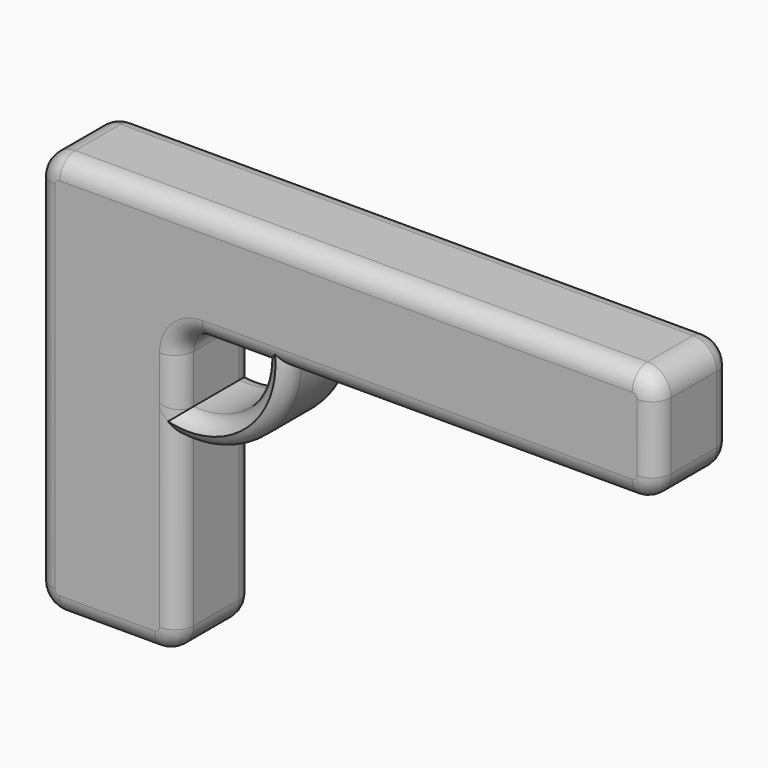
from build123d import *

# Parameters (mm, degrees)
F1_DEPTH      = 12.7
F2_T1_DEPTH   = 153.2337951016
F2_T3_DEPTH   = 95.3043418229
F2_T5_DEPTH   = 25.4
F2_T7_DEPTH   = 17.9600145107
F2_T10_ANGLE  = 90
F2_T12_ANGLE  = 90
F2_T14_ANGLE  = 90
F2_T18_DEPTH  = 58.0173112184
F2_S19_R      = 26.289
F2_T20_DEPTH  = 31
F2_T24_DEPTH  = 58.0173112184
F2_S25_R      = 20.32
F2_T26_DEPTH  = 31
F2_T30_ANGLE  = 149.8775603064
F2_T36_DEPTH  = 105.3526159376
F2_S37_R      = 20.32
F2_T38_DEPTH  = 54
F2_T42_DEPTH  = 105.3526159376
F2_S43_R      = 26.289
F2_T44_DEPTH  = 54
F2_T46_ANGLE  = 90
F2_T48_ANGLE  = 90
F2_T52_ANGLE  = 165.3398529119
F2_T58_DEPTH  = 25.6770160938
F2_S59_R      = 26.289
F2_T60_DEPTH  = 15
F2_T64_DEPTH  = 25.6770160938
F2_S65_R      = 20.32
F2_T66_DEPTH  = 15
F2_T68_ANGLE  = 90
F2_T72_DEPTH  = 28.831179164
F2_S73_R      = 20.32
F2_T74_DEPTH  = 16
F2_T78_DEPTH  = 28.831179164
F2_S79_R      = 26.289
F2_T80_DEPTH  = 16
F2_T82_ANGLE  = 90
F2_T84_ANGLE  = 90
F2_T86_ANGLE  = 90
F2_T90_DEPTH  = 58.0173112184
F2_S91_R      = 26.289
F2_T92_DEPTH  = 31
F2_T96_DEPTH  = 58.0173112184
F2_S97_R      = 20.32
F2_T98_DEPTH  = 31
F2_T102_ANGLE = 149.8775603064
F2_T108_DEPTH = 105.3526159376
F2_S109_R     = 20.32
F2_T110_DEPTH = 54
F2_T114_DEPTH = 105.3526159376
F2_S115_R     = 26.289
F2_T116_DEPTH = 54
F2_T118_ANGLE = 90
F2_T120_ANGLE = 90
F2_T124_ANGLE = 165.3398529119
F2_T130_DEPTH = 25.6770160938
F2_S131_R     = 26.289
F2_T132_DEPTH = 15
F2_T136_DEPTH = 25.6770160938
F2_S137_R     = 20.32
F2_T138_DEPTH = 15
F2_T140_ANGLE = 90
F2_T144_DEPTH = 28.831179164
F2_S145_R     = 20.32
F2_T146_DEPTH = 16
F2_T150_DEPTH = 28.831179164
F2_S151_R     = 26.289
F2_T152_DEPTH = 16
F2_T157_ANGLE = 149.8775603064
F2_T161_DEPTH = 58.0173112184
F2_S162_R     = 26.289
F2_T163_DEPTH = 31
F2_S164_R     = 20.32
F2_T165_DEPTH = 31
F2_T171_DEPTH = 105.3526159376
F2_S172_R     = 26.289
F2_T173_DEPTH = 54
F2_S174_R     = 20.32
F2_T175_DEPTH = 54
F2_T178_ANGLE = 149.8775603064
F2_T185_ANGLE = 165.3398529119
F2_T189_DEPTH = 28.831179164
F2_S190_R     = 26.289
F2_T191_DEPTH = 16
F2_S192_R     = 20.32
F2_T193_DEPTH = 16
F2_T199_ANGLE = 165.3398529119
F2_T203_DEPTH = 25.6770160938
F2_S204_R     = 26.289
F2_T205_DEPTH = 15
F2_S206_R     = 20.32
F2_T207_DEPTH = 15
F2_T213_ANGLE = 149.8775603064
F2_T217_DEPTH = 58.0173112184
F2_S218_R     = 26.289
F2_T219_DEPTH = 31
F2_S220_R     = 20.32
F2_T221_DEPTH = 31
F2_T227_DEPTH = 105.3526159376
F2_S228_R     = 26.289
F2_T229_DEPTH = 54
F2_S230_R     = 20.32
F2_T231_DEPTH = 54
F2_T234_ANGLE = 149.8775603064
F2_T241_DEPTH = 28.831179164
F2_S242_R     = 26.289
F2_T243_DEPTH = 16
F2_S244_R     = 20.32
F2_T245_DEPTH = 16
F2_T248_ANGLE = 165.3398529119
F2_T255_DEPTH = 25.6770160938
F2_S256_R     = 26.289
F2_T257_DEPTH = 15
F2_S258_R     = 20.32
F2_T259_DEPTH = 15
F2_T262_ANGLE = 165.3398529119


# Not quite as in the source:
# - a fillet or chamfer that OpenCascade refuses, or shapes differently, is made with other operations: its cross-section is extruded or revolved along the edge and cut away or added


with BuildPart() as f1:
    # F0 (on Front) → F1 (new body, symmetric)
    with BuildSketch(Plane.XZ):
        with BuildLine():
            Line((-31.75, -76.2), (-6.35, -76.2))
            ThreePointArc((-6.35, -76.2), (-1.8598719395, -74.3401280605), (0, -69.85))
            Line((0, -69.85), (0, -24.5326887816))
            ThreePointArc((0, -24.5326887816), (20.0309214376, -17.9992996084), (28.831179164, 1.1443273122))
            Line((28.831179164, 1.1443273122), (121.4837951016, 1.1443273122))
            ThreePointArc((121.4837951016, 1.1443273122), (125.9739231621, 3.0041992516), (127.8337951016, 7.4943273122))
            Line((127.8337951016, 7.4943273122), (127.8337951016, 25.4543418229))
            ThreePointArc((127.8337951016, 25.4543418229), (125.9739231621, 29.9444698834), (121.4837951016, 31.8043418229))
            Line((121.4837951016, 31.8043418229), (-31.75, 31.8043418229))
            ThreePointArc((-31.75, 31.8043418229), (-36.2401280605, 29.9444698834), (-38.1, 25.4543418229))
            Line((-38.1, 25.4543418229), (-38.1, -69.85))
            ThreePointArc((-38.1, -69.85), (-36.2401280605, -74.3401280605), (-31.75, -76.2))
        make_face()
        with BuildLine():
            Line((0, -18.1826887816), (0, -5.2056726878))
            ThreePointArc((0, -5.2056726878), (1.8598719395, -0.7155446273), (6.35, 1.1443273122))
            Line((6.35, 1.1443273122), (22.481179164, 1.1443273122))
            ThreePointArc((22.481179164, 1.1443273122), (15.4268166396, -13.3885987579), (0, -18.1826887816))
        make_face(mode=Mode.SUBTRACT)
    extrude(amount=F1_DEPTH, both=True)

    # F2: fillet of radius 5.08 on 32 edges, made by hand

    # F2_s2 → F2_t1 (cut)
    with BuildSketch(Plane.YZ.offset(-31.75)):
        with BuildLine():
            ThreePointArc((-7.62, 31.8043418229), (-11.2121024484, 30.3164442713), (-12.7, 26.7243418229))
            Line((-12.7, 26.7243418229), (-12.7, 31.8043418229))
            Line((-12.7, 31.8043418229), (-7.62, 31.8043418229))
        make_face()
        with BuildLine():
            ThreePointArc((7.62, 31.8043418229), (11.2121024484, 30.3164442713), (12.7, 26.7243418229))
            Line((12.7, 26.7243418229), (12.7, 31.8043418229))
            Line((12.7, 31.8043418229), (7.62, 31.8043418229))
        make_face()
    extrude(amount=F2_T1_DEPTH, mode=Mode.SUBTRACT)

    # F2_s4 → F2_t3 (cut)
    with BuildSketch(Plane.XY.offset(-69.85)):
        with BuildLine():
            ThreePointArc((-38.1, -7.62), (-36.6121024484, -11.2121024484), (-33.02, -12.7))
            Line((-33.02, -12.7), (-38.1, -12.7))
            Line((-38.1, -12.7), (-38.1, -7.62))
        make_face()
        with BuildLine():
            ThreePointArc((-38.1, 7.62), (-36.6121024484, 11.2121024484), (-33.02, 12.7))
            Line((-33.02, 12.7), (-38.1, 12.7))
            Line((-38.1, 12.7), (-38.1, 7.62))
        make_face()
    extrude(amount=F2_T3_DEPTH, mode=Mode.SUBTRACT)

    # F2_s6 → F2_t5 (cut)
    with BuildSketch(Plane.YZ.offset(-31.75)):
        with BuildLine():
            ThreePointArc((-7.62, -76.2), (-11.2121024484, -74.7121024484), (-12.7, -71.12))
            Line((-12.7, -71.12), (-12.7, -76.2))
            Line((-12.7, -76.2), (-7.62, -76.2))
        make_face()
        with BuildLine():
            ThreePointArc((7.62, -76.2), (11.2121024484, -74.7121024484), (12.7, -71.12))
            Line((12.7, -71.12), (12.7, -76.2))
            Line((12.7, -76.2), (7.62, -76.2))
        make_face()
    extrude(amount=F2_T5_DEPTH, mode=Mode.SUBTRACT)

    # F2_s8 → F2_t7 (cut)
    with BuildSketch(Plane.XY.offset(7.4943273122)):
        with BuildLine():
            ThreePointArc((127.8337951016, -7.62), (126.34589755, -11.2121024484), (122.7537951016, -12.7))
            Line((122.7537951016, -12.7), (127.8337951016, -12.7))
            Line((127.8337951016, -12.7), (127.8337951016, -7.62))
        make_face()
        with BuildLine():
            ThreePointArc((127.8337951016, 7.62), (126.34589755, 11.2121024484), (122.7537951016, 12.7))
            Line((122.7537951016, 12.7), (127.8337951016, 12.7))
            Line((127.8337951016, 12.7), (127.8337951016, 7.62))
        make_face()
    extrude(amount=F2_T7_DEPTH, mode=Mode.SUBTRACT)

    # F2_s9 → F2_t10 (revolve, cut)
    with BuildSketch(Plane.YZ.offset(-31.75)):
        with BuildLine():
            ThreePointArc((-12.7, 26.7243418229), (-11.2121024484, 30.3164442713), (-7.62, 31.8043418229))
            Line((-7.62, 31.8043418229), (-12.7, 31.8043418229))
            Line((-12.7, 31.8043418229), (-12.7, 26.7243418229))
        make_face()
    revolve(axis=Axis((-31.75, -12.7, 25.4543418229), (0, -1, 0)), revolution_arc=F2_T10_ANGLE, mode=Mode.SUBTRACT)

    # F2_s11 → F2_t12 (revolve, cut)
    with BuildSketch(Plane.XY.offset(-69.85)):
        with BuildLine():
            ThreePointArc((-38.1, -7.62), (-36.6121024484, -11.2121024484), (-33.02, -12.7))
            Line((-33.02, -12.7), (-38.1, -12.7))
            Line((-38.1, -12.7), (-38.1, -7.62))
        make_face()
    revolve(axis=Axis((-31.75, -12.7, -69.85), (0, -1, 0)), revolution_arc=F2_T12_ANGLE, mode=Mode.SUBTRACT)

    # F2_s13 → F2_t14 (revolve, cut)
    with BuildSketch(Plane.YZ.offset(-6.35)):
        with BuildLine():
            ThreePointArc((-7.62, -76.2), (-11.2121024484, -74.7121024484), (-12.7, -71.12))
            Line((-12.7, -71.12), (-12.7, -76.2))
            Line((-12.7, -76.2), (-7.62, -76.2))
        make_face()
    revolve(axis=Axis((-6.35, -12.7, -69.85), (0, -1, 0)), revolution_arc=F2_T14_ANGLE, mode=Mode.SUBTRACT)


with BuildPart() as f2_tool16:
    # F2_s17 → F2_t18 (new body)
    with BuildSketch(Plane.XY.offset(-69.85)):
        with BuildLine():
            ThreePointArc((0, -7.62), (-1.4878975516, -11.2121024484), (-5.08, -12.7))
            Line((-5.08, -12.7), (0, -12.7))
            Line((0, -12.7), (0, -7.62))
        make_face()
    extrude(amount=F2_T18_DEPTH)

    # F2_s19 → F2_t20 (cut, symmetric)
    with BuildSketch(Plane.XZ.offset(10.2)):
        with Locations((2.5467151815, 1.6326654637)):
            Circle(F2_S19_R)
    extrude(amount=F2_T20_DEPTH, both=True, mode=Mode.SUBTRACT)


with BuildPart() as f1_1:
    add(f1.part)

    # F2_t15: cut F2_tool16
    add(f2_tool16.part, mode=Mode.SUBTRACT)


with BuildPart() as f2_tool22:
    # F2_s23 → F2_t24 (new body)
    with BuildSketch(Plane.XY.offset(-69.85)):
        with BuildLine():
            ThreePointArc((0, -7.62), (-1.4878975516, -11.2121024484), (-5.08, -12.7))
            Line((-5.08, -12.7), (0, -12.7))
            Line((0, -12.7), (0, -7.62))
        make_face()
    extrude(amount=F2_T24_DEPTH)

    # F2_s25 → F2_t26 (intersect, symmetric)
    with BuildSketch(Plane.XZ.offset(10.2)):
        with Locations((2.1800572993, 2.0200276241)):
            Circle(F2_S25_R)
    extrude(amount=F2_T26_DEPTH, both=True, mode=Mode.INTERSECT)


with BuildPart() as f1_2:
    add(f1_1.part)

    # F2_t21: cut F2_tool22
    add(f2_tool22.part, mode=Mode.SUBTRACT)


with BuildPart() as f2_tool28:
    # F2_s29 → F2_t30 (revolve)
    with BuildSketch(Plane(origin=(1.0324526072, 0, -0.6769199165), x_dir=(0, 1, 0), z_dir=(-0.8362808351, 0, 0.5483013449))):
        with BuildLine():
            ThreePointArc((-7.62, 23.5272658034), (-11.2121024484, 22.0393682518), (-12.7, 18.4472658034))
            Line((-12.7, 18.4472658034), (-12.7, 23.5272658034))
            Line((-12.7, 23.5272658034), (-7.62, 23.5272658034))
        make_face()
    revolve(axis=Axis((2.5467151815, -12.7, 1.6326654637), (0, -1, 0)), revolution_arc=F2_T30_ANGLE)

    split(bisect_by=Plane.XY.offset(1.1443273122), keep=Keep.BOTTOM)

    split(bisect_by=Plane.YZ, keep=Keep.TOP)


with BuildPart() as f1_3:
    add(f1_2.part)

    # F2_t27: cut F2_tool28
    add(f2_tool28.part, mode=Mode.SUBTRACT)


with BuildPart() as f2_tool34:
    # F2_s35 → F2_t36 (new body)
    with BuildSketch(Plane.YZ.offset(16.131179164)):
        with BuildLine():
            ThreePointArc((-7.62, 1.1443273122), (-11.2121024484, 2.6322248637), (-12.7, 6.2243273122))
            Line((-12.7, 6.2243273122), (-12.7, 1.1443273122))
            Line((-12.7, 1.1443273122), (-7.62, 1.1443273122))
        make_face()
    extrude(amount=F2_T36_DEPTH)

    # F2_s37 → F2_t38 (intersect, symmetric)
    with BuildSketch(Plane.XZ.offset(10.2)):
        with Locations((2.1800572993, 2.0200276241)):
            Circle(F2_S37_R)
    extrude(amount=F2_T38_DEPTH, both=True, mode=Mode.INTERSECT)


with BuildPart() as f1_4:
    add(f1_3.part)

    # F2_t33: cut F2_tool34
    add(f2_tool34.part, mode=Mode.SUBTRACT)


with BuildPart() as f2_tool40:
    # F2_s41 → F2_t42 (new body)
    with BuildSketch(Plane.YZ.offset(16.131179164)):
        with BuildLine():
            ThreePointArc((-7.62, 1.1443273122), (-11.2121024484, 2.6322248637), (-12.7, 6.2243273122))
            Line((-12.7, 6.2243273122), (-12.7, 1.1443273122))
            Line((-12.7, 1.1443273122), (-7.62, 1.1443273122))
        make_face()
    extrude(amount=F2_T42_DEPTH)

    # F2_s43 → F2_t44 (cut, symmetric)
    with BuildSketch(Plane.XZ.offset(10.2)):
        with Locations((2.5467151815, 1.6326654637)):
            Circle(F2_S43_R)
    extrude(amount=F2_T44_DEPTH, both=True, mode=Mode.SUBTRACT)


with BuildPart() as f1_5:
    add(f1_4.part)

    # F2_t39: cut F2_tool40
    add(f2_tool40.part, mode=Mode.SUBTRACT)

    # F2_s45 → F2_t46 (revolve, cut)
    with BuildSketch(Plane.YZ.offset(121.4837951016)):
        with BuildLine():
            ThreePointArc((-7.62, 1.1443273122), (-11.2121024484, 2.6322248637), (-12.7, 6.2243273122))
            Line((-12.7, 6.2243273122), (-12.7, 1.1443273122))
            Line((-12.7, 1.1443273122), (-7.62, 1.1443273122))
        make_face()
    revolve(axis=Axis((121.4837951016, -12.7, 7.4943273122), (0, -1, 0)), revolution_arc=F2_T46_ANGLE, mode=Mode.SUBTRACT)

    # F2_s47 → F2_t48 (revolve, cut)
    with BuildSketch(Plane.XY.offset(25.4543418229)):
        with BuildLine():
            ThreePointArc((127.8337951016, -7.62), (126.34589755, -11.2121024484), (122.7537951016, -12.7))
            Line((122.7537951016, -12.7), (127.8337951016, -12.7))
            Line((127.8337951016, -12.7), (127.8337951016, -7.62))
        make_face()
    revolve(axis=Axis((121.4837951016, -12.7, 25.4543418229), (0, -1, 0)), revolution_arc=F2_T48_ANGLE, mode=Mode.SUBTRACT)


with BuildPart() as f2_tool50:
    # F2_s51 → F2_t52 (revolve)
    with BuildSketch(Plane(origin=(-0.2686553541, 0, 0.4081266668), x_dir=(0, 1, 0), z_dir=(-0.5498321217, 0, 0.835275187))):
        with BuildLine():
            ThreePointArc((-12.7, -28.3316238427), (-11.2121024484, -24.7395213943), (-7.62, -23.2516238427))
            Line((-7.62, -23.2516238427), (-12.7, -23.2516238427))
            Line((-12.7, -23.2516238427), (-12.7, -28.3316238427))
        make_face()
    revolve(axis=Axis((2.1800572993, -12.7, 2.0200276241), (0, 1, 0)), revolution_arc=F2_T52_ANGLE)

    split(bisect_by=Plane.XY.offset(1.1443273122), keep=Keep.BOTTOM)

    split(bisect_by=Plane.YZ, keep=Keep.TOP)


with BuildPart() as f1_6:
    add(f1_5.part)

    # F2_t49: cut F2_tool50
    add(f2_tool50.part, mode=Mode.SUBTRACT)


with BuildPart() as f2_tool56:
    # F2_s57 → F2_t58 (new body)
    with BuildSketch(Plane.XY.offset(-30.8826887816)):
        with BuildLine():
            ThreePointArc((-5.08, -12.7), (-1.4878975516, -11.2121024484), (0, -7.62))
            Line((0, -7.62), (0, -12.7))
            Line((0, -12.7), (-5.08, -12.7))
        make_face()
    extrude(amount=F2_T58_DEPTH)

    # F2_s59 → F2_t60 (cut, symmetric)
    with BuildSketch(Plane.XZ.offset(10.2)):
        with Locations((2.5467151815, 1.6326654637)):
            Circle(F2_S59_R)
    extrude(amount=F2_T60_DEPTH, both=True, mode=Mode.SUBTRACT)


with BuildPart() as f1_7:
    add(f1_6.part)

    # F2_t55: cut F2_tool56
    add(f2_tool56.part, mode=Mode.SUBTRACT)


with BuildPart() as f2_tool62:
    # F2_s63 → F2_t64 (new body)
    with BuildSketch(Plane.XY.offset(-30.8826887816)):
        with BuildLine():
            ThreePointArc((-5.08, -12.7), (-1.4878975516, -11.2121024484), (0, -7.62))
            Line((0, -7.62), (0, -12.7))
            Line((0, -12.7), (-5.08, -12.7))
        make_face()
    extrude(amount=F2_T64_DEPTH)

    # F2_s65 → F2_t66 (intersect, symmetric)
    with BuildSketch(Plane.XZ.offset(10.2)):
        with Locations((2.1800572993, 2.0200276241)):
            Circle(F2_S65_R)
    extrude(amount=F2_T66_DEPTH, both=True, mode=Mode.INTERSECT)


with BuildPart() as f1_8:
    add(f1_7.part)

    # F2_t61: cut F2_tool62
    add(f2_tool62.part, mode=Mode.SUBTRACT)

    # F2_s67 → F2_t68 (revolve, cut)
    with BuildSketch(Plane.XY.offset(-5.2056726878)):
        with BuildLine():
            ThreePointArc((-5.08, -12.7), (-1.4878975516, -11.2121024484), (0, -7.62))
            Line((0, -7.62), (0, -12.7))
            Line((0, -12.7), (-5.08, -12.7))
        make_face()
    revolve(axis=Axis((6.35, -12.7, -5.2056726878), (0, 1, 0)), revolution_arc=F2_T68_ANGLE, mode=Mode.SUBTRACT)


with BuildPart() as f2_tool70:
    # F2_s71 → F2_t72 (new body)
    with BuildSketch(Plane.YZ.offset(6.35)):
        with BuildLine():
            ThreePointArc((-12.7, 6.2243273122), (-11.2121024484, 2.6322248637), (-7.62, 1.1443273122))
            Line((-7.62, 1.1443273122), (-12.7, 1.1443273122))
            Line((-12.7, 1.1443273122), (-12.7, 6.2243273122))
        make_face()
    extrude(amount=F2_T72_DEPTH)

    # F2_s73 → F2_t74 (intersect, symmetric)
    with BuildSketch(Plane.XZ.offset(10.2)):
        with Locations((2.1800572993, 2.0200276241)):
            Circle(F2_S73_R)
    extrude(amount=F2_T74_DEPTH, both=True, mode=Mode.INTERSECT)


with BuildPart() as f1_9:
    add(f1_8.part)

    # F2_t69: cut F2_tool70
    add(f2_tool70.part, mode=Mode.SUBTRACT)


with BuildPart() as f2_tool76:
    # F2_s77 → F2_t78 (new body)
    with BuildSketch(Plane.YZ.offset(6.35)):
        with BuildLine():
            ThreePointArc((-12.7, 6.2243273122), (-11.2121024484, 2.6322248637), (-7.62, 1.1443273122))
            Line((-7.62, 1.1443273122), (-12.7, 1.1443273122))
            Line((-12.7, 1.1443273122), (-12.7, 6.2243273122))
        make_face()
    extrude(amount=F2_T78_DEPTH)

    # F2_s79 → F2_t80 (cut, symmetric)
    with BuildSketch(Plane.XZ.offset(10.2)):
        with Locations((2.5467151815, 1.6326654637)):
            Circle(F2_S79_R)
    extrude(amount=F2_T80_DEPTH, both=True, mode=Mode.SUBTRACT)


with BuildPart() as f1_10:
    add(f1_9.part)

    # F2_t75: cut F2_tool76
    add(f2_tool76.part, mode=Mode.SUBTRACT)

    # F2_s81 → F2_t82 (revolve, cut)
    with BuildSketch(Plane.YZ.offset(-31.75)):
        with BuildLine():
            ThreePointArc((7.62, 31.8043418229), (11.2121024484, 30.3164442713), (12.7, 26.7243418229))
            Line((12.7, 26.7243418229), (12.7, 31.8043418229))
            Line((12.7, 31.8043418229), (7.62, 31.8043418229))
        make_face()
    revolve(axis=Axis((-31.75, 12.7, 25.4543418229), (0, -1, 0)), revolution_arc=F2_T82_ANGLE, mode=Mode.SUBTRACT)

    # F2_s83 → F2_t84 (revolve, cut)
    with BuildSketch(Plane.XY.offset(-69.85)):
        with BuildLine():
            ThreePointArc((-38.1, 7.62), (-36.6121024484, 11.2121024484), (-33.02, 12.7))
            Line((-33.02, 12.7), (-38.1, 12.7))
            Line((-38.1, 12.7), (-38.1, 7.62))
        make_face()
    revolve(axis=Axis((-31.75, 12.7, -69.85), (0, -1, 0)), revolution_arc=F2_T84_ANGLE, mode=Mode.SUBTRACT)

    # F2_s85 → F2_t86 (revolve, cut)
    with BuildSketch(Plane.YZ.offset(-6.35)):
        with BuildLine():
            ThreePointArc((7.62, -76.2), (11.2121024484, -74.7121024484), (12.7, -71.12))
            Line((12.7, -71.12), (12.7, -76.2))
            Line((12.7, -76.2), (7.62, -76.2))
        make_face()
    revolve(axis=Axis((-6.35, 12.7, -69.85), (0, -1, 0)), revolution_arc=F2_T86_ANGLE, mode=Mode.SUBTRACT)


with BuildPart() as f2_tool88:
    # F2_s89 → F2_t90 (new body)
    with BuildSketch(Plane.XY.offset(-69.85)):
        with BuildLine():
            ThreePointArc((0, 7.62), (-1.4878975516, 11.2121024484), (-5.08, 12.7))
            Line((-5.08, 12.7), (0, 12.7))
            Line((0, 12.7), (0, 7.62))
        make_face()
    extrude(amount=F2_T90_DEPTH)

    # F2_s91 → F2_t92 (cut, symmetric)
    with BuildSketch(Plane.XZ.offset(-10.2)):
        with Locations((2.5467151815, 1.6326654637)):
            Circle(F2_S91_R)
    extrude(amount=F2_T92_DEPTH, both=True, mode=Mode.SUBTRACT)


with BuildPart() as f1_11:
    add(f1_10.part)

    # F2_t87: cut F2_tool88
    add(f2_tool88.part, mode=Mode.SUBTRACT)


with BuildPart() as f2_tool94:
    # F2_s95 → F2_t96 (new body)
    with BuildSketch(Plane.XY.offset(-69.85)):
        with BuildLine():
            ThreePointArc((0, 7.62), (-1.4878975516, 11.2121024484), (-5.08, 12.7))
            Line((-5.08, 12.7), (0, 12.7))
            Line((0, 12.7), (0, 7.62))
        make_face()
    extrude(amount=F2_T96_DEPTH)

    # F2_s97 → F2_t98 (intersect, symmetric)
    with BuildSketch(Plane.XZ.offset(-10.2)):
        with Locations((2.1800572993, 2.0200276241)):
            Circle(F2_S97_R)
    extrude(amount=F2_T98_DEPTH, both=True, mode=Mode.INTERSECT)


with BuildPart() as f1_12:
    add(f1_11.part)

    # F2_t93: cut F2_tool94
    add(f2_tool94.part, mode=Mode.SUBTRACT)


with BuildPart() as f2_tool100:
    # F2_s101 → F2_t102 (revolve)
    with BuildSketch(Plane(origin=(1.0324526072, 0, -0.6769199165), x_dir=(0, 1, 0), z_dir=(-0.8362808351, 0, 0.5483013449))):
        with BuildLine():
            ThreePointArc((7.62, 23.5272658034), (11.2121024484, 22.0393682518), (12.7, 18.4472658034))
            Line((12.7, 18.4472658034), (12.7, 23.5272658034))
            Line((12.7, 23.5272658034), (7.62, 23.5272658034))
        make_face()
    revolve(axis=Axis((2.5467151815, 12.7, 1.6326654637), (0, -1, 0)), revolution_arc=F2_T102_ANGLE)

    split(bisect_by=Plane.XY.offset(1.1443273122), keep=Keep.BOTTOM)

    split(bisect_by=Plane.YZ, keep=Keep.TOP)


with BuildPart() as f1_13:
    add(f1_12.part)

    # F2_t99: cut F2_tool100
    add(f2_tool100.part, mode=Mode.SUBTRACT)


with BuildPart() as f2_tool106:
    # F2_s107 → F2_t108 (new body)
    with BuildSketch(Plane.YZ.offset(16.131179164)):
        with BuildLine():
            ThreePointArc((7.62, 1.1443273122), (11.2121024484, 2.6322248637), (12.7, 6.2243273122))
            Line((12.7, 6.2243273122), (12.7, 1.1443273122))
            Line((12.7, 1.1443273122), (7.62, 1.1443273122))
        make_face()
    extrude(amount=F2_T108_DEPTH)

    # F2_s109 → F2_t110 (intersect, symmetric)
    with BuildSketch(Plane.XZ.offset(-10.2)):
        with Locations((2.1800572993, 2.0200276241)):
            Circle(F2_S109_R)
    extrude(amount=F2_T110_DEPTH, both=True, mode=Mode.INTERSECT)


with BuildPart() as f1_14:
    add(f1_13.part)

    # F2_t105: cut F2_tool106
    add(f2_tool106.part, mode=Mode.SUBTRACT)


with BuildPart() as f2_tool112:
    # F2_s113 → F2_t114 (new body)
    with BuildSketch(Plane.YZ.offset(16.131179164)):
        with BuildLine():
            ThreePointArc((7.62, 1.1443273122), (11.2121024484, 2.6322248637), (12.7, 6.2243273122))
            Line((12.7, 6.2243273122), (12.7, 1.1443273122))
            Line((12.7, 1.1443273122), (7.62, 1.1443273122))
        make_face()
    extrude(amount=F2_T114_DEPTH)

    # F2_s115 → F2_t116 (cut, symmetric)
    with BuildSketch(Plane.XZ.offset(-10.2)):
        with Locations((2.5467151815, 1.6326654637)):
            Circle(F2_S115_R)
    extrude(amount=F2_T116_DEPTH, both=True, mode=Mode.SUBTRACT)


with BuildPart() as f1_15:
    add(f1_14.part)

    # F2_t111: cut F2_tool112
    add(f2_tool112.part, mode=Mode.SUBTRACT)

    # F2_s117 → F2_t118 (revolve, cut)
    with BuildSketch(Plane.YZ.offset(121.4837951016)):
        with BuildLine():
            ThreePointArc((7.62, 1.1443273122), (11.2121024484, 2.6322248637), (12.7, 6.2243273122))
            Line((12.7, 6.2243273122), (12.7, 1.1443273122))
            Line((12.7, 1.1443273122), (7.62, 1.1443273122))
        make_face()
    revolve(axis=Axis((121.4837951016, 12.7, 7.4943273122), (0, -1, 0)), revolution_arc=F2_T118_ANGLE, mode=Mode.SUBTRACT)

    # F2_s119 → F2_t120 (revolve, cut)
    with BuildSketch(Plane.XY.offset(25.4543418229)):
        with BuildLine():
            ThreePointArc((127.8337951016, 7.62), (126.34589755, 11.2121024484), (122.7537951016, 12.7))
            Line((122.7537951016, 12.7), (127.8337951016, 12.7))
            Line((127.8337951016, 12.7), (127.8337951016, 7.62))
        make_face()
    revolve(axis=Axis((121.4837951016, 12.7, 25.4543418229), (0, -1, 0)), revolution_arc=F2_T120_ANGLE, mode=Mode.SUBTRACT)


with BuildPart() as f2_tool122:
    # F2_s123 → F2_t124 (revolve)
    with BuildSketch(Plane(origin=(-0.2686553541, 0, 0.4081266668), x_dir=(0, 1, 0), z_dir=(-0.5498321217, 0, 0.835275187))):
        with BuildLine():
            ThreePointArc((7.62, -23.2516238427), (11.2121024484, -24.7395213943), (12.7, -28.3316238427))
            Line((12.7, -28.3316238427), (12.7, -23.2516238427))
            Line((12.7, -23.2516238427), (7.62, -23.2516238427))
        make_face()
    revolve(axis=Axis((2.1800572993, 12.7, 2.0200276241), (0, 1, 0)), revolution_arc=F2_T124_ANGLE)

    split(bisect_by=Plane.XY.offset(1.1443273122), keep=Keep.BOTTOM)

    split(bisect_by=Plane.YZ, keep=Keep.TOP)


with BuildPart() as f1_16:
    add(f1_15.part)

    # F2_t121: cut F2_tool122
    add(f2_tool122.part, mode=Mode.SUBTRACT)


with BuildPart() as f2_tool128:
    # F2_s129 → F2_t130 (new body)
    with BuildSketch(Plane.XY.offset(-30.8826887816)):
        with BuildLine():
            ThreePointArc((0, 7.62), (-1.4878975516, 11.2121024484), (-5.08, 12.7))
            Line((-5.08, 12.7), (0, 12.7))
            Line((0, 12.7), (0, 7.62))
        make_face()
    extrude(amount=F2_T130_DEPTH)

    # F2_s131 → F2_t132 (cut, symmetric)
    with BuildSketch(Plane.XZ.offset(-10.2)):
        with Locations((2.5467151815, 1.6326654637)):
            Circle(F2_S131_R)
    extrude(amount=F2_T132_DEPTH, both=True, mode=Mode.SUBTRACT)


with BuildPart() as f1_17:
    add(f1_16.part)

    # F2_t127: cut F2_tool128
    add(f2_tool128.part, mode=Mode.SUBTRACT)


with BuildPart() as f2_tool134:
    # F2_s135 → F2_t136 (new body)
    with BuildSketch(Plane.XY.offset(-30.8826887816)):
        with BuildLine():
            ThreePointArc((0, 7.62), (-1.4878975516, 11.2121024484), (-5.08, 12.7))
            Line((-5.08, 12.7), (0, 12.7))
            Line((0, 12.7), (0, 7.62))
        make_face()
    extrude(amount=F2_T136_DEPTH)

    # F2_s137 → F2_t138 (intersect, symmetric)
    with BuildSketch(Plane.XZ.offset(-10.2)):
        with Locations((2.1800572993, 2.0200276241)):
            Circle(F2_S137_R)
    extrude(amount=F2_T138_DEPTH, both=True, mode=Mode.INTERSECT)


with BuildPart() as f1_18:
    add(f1_17.part)

    # F2_t133: cut F2_tool134
    add(f2_tool134.part, mode=Mode.SUBTRACT)

    # F2_s139 → F2_t140 (revolve, cut)
    with BuildSketch(Plane.XY.offset(-5.2056726878)):
        with BuildLine():
            ThreePointArc((0, 7.62), (-1.4878975516, 11.2121024484), (-5.08, 12.7))
            Line((-5.08, 12.7), (0, 12.7))
            Line((0, 12.7), (0, 7.62))
        make_face()
    revolve(axis=Axis((6.35, 12.7, -5.2056726878), (0, 1, 0)), revolution_arc=F2_T140_ANGLE, mode=Mode.SUBTRACT)


with BuildPart() as f2_tool142:
    # F2_s143 → F2_t144 (new body)
    with BuildSketch(Plane.YZ.offset(6.35)):
        with BuildLine():
            ThreePointArc((7.62, 1.1443273122), (11.2121024484, 2.6322248637), (12.7, 6.2243273122))
            Line((12.7, 6.2243273122), (12.7, 1.1443273122))
            Line((12.7, 1.1443273122), (7.62, 1.1443273122))
        make_face()
    extrude(amount=F2_T144_DEPTH)

    # F2_s145 → F2_t146 (intersect, symmetric)
    with BuildSketch(Plane.XZ.offset(-10.2)):
        with Locations((2.1800572993, 2.0200276241)):
            Circle(F2_S145_R)
    extrude(amount=F2_T146_DEPTH, both=True, mode=Mode.INTERSECT)


with BuildPart() as f1_19:
    add(f1_18.part)

    # F2_t141: cut F2_tool142
    add(f2_tool142.part, mode=Mode.SUBTRACT)


with BuildPart() as f2_tool148:
    # F2_s149 → F2_t150 (new body)
    with BuildSketch(Plane.YZ.offset(6.35)):
        with BuildLine():
            ThreePointArc((7.62, 1.1443273122), (11.2121024484, 2.6322248637), (12.7, 6.2243273122))
            Line((12.7, 6.2243273122), (12.7, 1.1443273122))
            Line((12.7, 1.1443273122), (7.62, 1.1443273122))
        make_face()
    extrude(amount=F2_T150_DEPTH)

    # F2_s151 → F2_t152 (cut, symmetric)
    with BuildSketch(Plane.XZ.offset(-10.2)):
        with Locations((2.5467151815, 1.6326654637)):
            Circle(F2_S151_R)
    extrude(amount=F2_T152_DEPTH, both=True, mode=Mode.SUBTRACT)


with BuildPart() as f1_20:
    add(f1_19.part)

    # F2_t147: cut F2_tool148
    add(f2_tool148.part, mode=Mode.SUBTRACT)


with BuildPart() as f2_tool155:
    # F2_s156 → F2_t157 (revolve)
    with BuildSketch(Plane(origin=(1.0324526072, 0, -0.6769199165), x_dir=(0, 1, 0), z_dir=(-0.8362808351, 0, 0.5483013449))):
        with BuildLine():
            ThreePointArc((-7.62, 23.5272658034), (-11.2121024484, 22.0393682518), (-12.7, 18.4472658034))
            Line((-12.7, 18.4472658034), (-12.7, 23.5272658034))
            Line((-12.7, 23.5272658034), (-7.62, 23.5272658034))
        make_face()
    revolve(axis=Axis((2.5467151815, -12.7, 1.6326654637), (0, -1, 0)), revolution_arc=F2_T157_ANGLE)

    split(bisect_by=Plane.YZ, keep=Keep.BOTTOM)


with BuildPart() as f2_tool159:
    # F2_s160 → F2_t161 (new body)
    with BuildSketch(Plane.XY.offset(-69.85)):
        with BuildLine():
            ThreePointArc((0, -7.62), (-1.4878975516, -11.2121024484), (-5.08, -12.7))
            Line((-5.08, -12.7), (0, -12.7))
            Line((0, -12.7), (0, -7.62))
        make_face()
    extrude(amount=F2_T161_DEPTH)

    # F2_s162 → F2_t163 (intersect, symmetric)
    with BuildSketch(Plane.XZ.offset(10.2)):
        with Locations((2.5467151815, 1.6326654637)):
            Circle(F2_S162_R)
    extrude(amount=F2_T163_DEPTH, both=True, mode=Mode.INTERSECT)

    # F2_s164 → F2_t165 (cut, symmetric)
    with BuildSketch(Plane.XZ.offset(10.2)):
        with Locations((2.1800572993, 2.0200276241)):
            Circle(F2_S164_R)
    extrude(amount=F2_T165_DEPTH, both=True, mode=Mode.SUBTRACT)


with BuildPart() as f2_tool155_1:
    add(f2_tool155.part)

    # F2_t166: intersect F2_tool159
    add(f2_tool159.part, mode=Mode.INTERSECT)


with BuildPart() as f1_21:
    add(f1_20.part)

    # F2_t153: cut F2_tool155
    add(f2_tool155_1.part, mode=Mode.SUBTRACT)


with BuildPart() as f2_tool169:
    # F2_s170 → F2_t171 (new body)
    with BuildSketch(Plane.YZ.offset(16.131179164)):
        with BuildLine():
            ThreePointArc((-7.62, 1.1443273122), (-11.2121024484, 2.6322248637), (-12.7, 6.2243273122))
            Line((-12.7, 6.2243273122), (-12.7, 1.1443273122))
            Line((-12.7, 1.1443273122), (-7.62, 1.1443273122))
        make_face()
    extrude(amount=F2_T171_DEPTH)

    # F2_s172 → F2_t173 (intersect, symmetric)
    with BuildSketch(Plane.XZ.offset(10.2)):
        with Locations((2.5467151815, 1.6326654637)):
            Circle(F2_S172_R)
    extrude(amount=F2_T173_DEPTH, both=True, mode=Mode.INTERSECT)

    # F2_s174 → F2_t175 (cut, symmetric)
    with BuildSketch(Plane.XZ.offset(10.2)):
        with Locations((2.1800572993, 2.0200276241)):
            Circle(F2_S174_R)
    extrude(amount=F2_T175_DEPTH, both=True, mode=Mode.SUBTRACT)


with BuildPart() as f2_tool176:
    # F2_s177 → F2_t178 (revolve)
    with BuildSketch(Plane(origin=(1.0324526072, 0, -0.6769199165), x_dir=(0, 1, 0), z_dir=(-0.8362808351, 0, 0.5483013449))):
        with BuildLine():
            ThreePointArc((-7.62, 23.5272658034), (-11.2121024484, 22.0393682518), (-12.7, 18.4472658034))
            Line((-12.7, 18.4472658034), (-12.7, 23.5272658034))
            Line((-12.7, 23.5272658034), (-7.62, 23.5272658034))
        make_face()
    revolve(axis=Axis((2.5467151815, -12.7, 1.6326654637), (0, -1, 0)), revolution_arc=F2_T178_ANGLE)

    split(bisect_by=Plane.XY.offset(1.1443273122), keep=Keep.TOP)


with BuildPart() as f2_tool169_1:
    add(f2_tool169.part)

    # F2_t180: intersect F2_tool176
    add(f2_tool176.part, mode=Mode.INTERSECT)


with BuildPart() as f1_22:
    add(f1_21.part)

    # F2_t167: cut F2_tool169
    add(f2_tool169_1.part, mode=Mode.SUBTRACT)


with BuildPart() as f2_tool183:
    # F2_s184 → F2_t185 (revolve)
    with BuildSketch(Plane(origin=(-0.2686553541, 0, 0.4081266668), x_dir=(0, 1, 0), z_dir=(-0.5498321217, 0, 0.835275187))):
        with BuildLine():
            ThreePointArc((-12.7, -28.3316238427), (-11.2121024484, -24.7395213943), (-7.62, -23.2516238427))
            Line((-7.62, -23.2516238427), (-12.7, -23.2516238427))
            Line((-12.7, -23.2516238427), (-12.7, -28.3316238427))
        make_face()
    revolve(axis=Axis((2.1800572993, -12.7, 2.0200276241), (0, 1, 0)), revolution_arc=F2_T185_ANGLE)

    split(bisect_by=Plane.XY.offset(1.1443273122), keep=Keep.TOP)


with BuildPart() as f2_tool187:
    # F2_s188 → F2_t189 (new body)
    with BuildSketch(Plane.YZ.offset(6.35)):
        with BuildLine():
            ThreePointArc((-12.7, 6.2243273122), (-11.2121024484, 2.6322248637), (-7.62, 1.1443273122))
            Line((-7.62, 1.1443273122), (-12.7, 1.1443273122))
            Line((-12.7, 1.1443273122), (-12.7, 6.2243273122))
        make_face()
    extrude(amount=F2_T189_DEPTH)

    # F2_s190 → F2_t191 (intersect, symmetric)
    with BuildSketch(Plane.XZ.offset(10.2)):
        with Locations((2.5467151815, 1.6326654637)):
            Circle(F2_S190_R)
    extrude(amount=F2_T191_DEPTH, both=True, mode=Mode.INTERSECT)

    # F2_s192 → F2_t193 (cut, symmetric)
    with BuildSketch(Plane.XZ.offset(10.2)):
        with Locations((2.1800572993, 2.0200276241)):
            Circle(F2_S192_R)
    extrude(amount=F2_T193_DEPTH, both=True, mode=Mode.SUBTRACT)


with BuildPart() as f2_tool183_1:
    add(f2_tool183.part)

    # F2_t194: intersect F2_tool187
    add(f2_tool187.part, mode=Mode.INTERSECT)


with BuildPart() as f1_23:
    add(f1_22.part)

    # F2_t181: cut F2_tool183
    add(f2_tool183_1.part, mode=Mode.SUBTRACT)


with BuildPart() as f2_tool197:
    # F2_s198 → F2_t199 (revolve)
    with BuildSketch(Plane(origin=(-0.2686553541, 0, 0.4081266668), x_dir=(0, 1, 0), z_dir=(-0.5498321217, 0, 0.835275187))):
        with BuildLine():
            ThreePointArc((-12.7, -28.3316238427), (-11.2121024484, -24.7395213943), (-7.62, -23.2516238427))
            Line((-7.62, -23.2516238427), (-12.7, -23.2516238427))
            Line((-12.7, -23.2516238427), (-12.7, -28.3316238427))
        make_face()
    revolve(axis=Axis((2.1800572993, -12.7, 2.0200276241), (0, 1, 0)), revolution_arc=F2_T199_ANGLE)

    split(bisect_by=Plane.YZ, keep=Keep.BOTTOM)


with BuildPart() as f2_tool201:
    # F2_s202 → F2_t203 (new body)
    with BuildSketch(Plane.XY.offset(-30.8826887816)):
        with BuildLine():
            ThreePointArc((-5.08, -12.7), (-1.4878975516, -11.2121024484), (0, -7.62))
            Line((0, -7.62), (0, -12.7))
            Line((0, -12.7), (-5.08, -12.7))
        make_face()
    extrude(amount=F2_T203_DEPTH)

    # F2_s204 → F2_t205 (intersect, symmetric)
    with BuildSketch(Plane.XZ.offset(10.2)):
        with Locations((2.5467151815, 1.6326654637)):
            Circle(F2_S204_R)
    extrude(amount=F2_T205_DEPTH, both=True, mode=Mode.INTERSECT)

    # F2_s206 → F2_t207 (cut, symmetric)
    with BuildSketch(Plane.XZ.offset(10.2)):
        with Locations((2.1800572993, 2.0200276241)):
            Circle(F2_S206_R)
    extrude(amount=F2_T207_DEPTH, both=True, mode=Mode.SUBTRACT)


with BuildPart() as f2_tool197_1:
    add(f2_tool197.part)

    # F2_t208: intersect F2_tool201
    add(f2_tool201.part, mode=Mode.INTERSECT)


with BuildPart() as f1_24:
    add(f1_23.part)

    # F2_t195: cut F2_tool197
    add(f2_tool197_1.part, mode=Mode.SUBTRACT)


with BuildPart() as f2_tool211:
    # F2_s212 → F2_t213 (revolve)
    with BuildSketch(Plane(origin=(1.0324526072, 0, -0.6769199165), x_dir=(0, 1, 0), z_dir=(-0.8362808351, 0, 0.5483013449))):
        with BuildLine():
            ThreePointArc((7.62, 23.5272658034), (11.2121024484, 22.0393682518), (12.7, 18.4472658034))
            Line((12.7, 18.4472658034), (12.7, 23.5272658034))
            Line((12.7, 23.5272658034), (7.62, 23.5272658034))
        make_face()
    revolve(axis=Axis((2.5467151815, 12.7, 1.6326654637), (0, -1, 0)), revolution_arc=F2_T213_ANGLE)

    split(bisect_by=Plane.YZ, keep=Keep.BOTTOM)


with BuildPart() as f2_tool215:
    # F2_s216 → F2_t217 (new body)
    with BuildSketch(Plane.XY.offset(-69.85)):
        with BuildLine():
            ThreePointArc((0, 7.62), (-1.4878975516, 11.2121024484), (-5.08, 12.7))
            Line((-5.08, 12.7), (0, 12.7))
            Line((0, 12.7), (0, 7.62))
        make_face()
    extrude(amount=F2_T217_DEPTH)

    # F2_s218 → F2_t219 (intersect, symmetric)
    with BuildSketch(Plane.XZ.offset(-10.2)):
        with Locations((2.5467151815, 1.6326654637)):
            Circle(F2_S218_R)
    extrude(amount=F2_T219_DEPTH, both=True, mode=Mode.INTERSECT)

    # F2_s220 → F2_t221 (cut, symmetric)
    with BuildSketch(Plane.XZ.offset(-10.2)):
        with Locations((2.1800572993, 2.0200276241)):
            Circle(F2_S220_R)
    extrude(amount=F2_T221_DEPTH, both=True, mode=Mode.SUBTRACT)


with BuildPart() as f2_tool211_1:
    add(f2_tool211.part)

    # F2_t222: intersect F2_tool215
    add(f2_tool215.part, mode=Mode.INTERSECT)


with BuildPart() as f1_25:
    add(f1_24.part)

    # F2_t209: cut F2_tool211
    add(f2_tool211_1.part, mode=Mode.SUBTRACT)


with BuildPart() as f2_tool225:
    # F2_s226 → F2_t227 (new body)
    with BuildSketch(Plane.YZ.offset(16.131179164)):
        with BuildLine():
            ThreePointArc((7.62, 1.1443273122), (11.2121024484, 2.6322248637), (12.7, 6.2243273122))
            Line((12.7, 6.2243273122), (12.7, 1.1443273122))
            Line((12.7, 1.1443273122), (7.62, 1.1443273122))
        make_face()
    extrude(amount=F2_T227_DEPTH)

    # F2_s228 → F2_t229 (intersect, symmetric)
    with BuildSketch(Plane.XZ.offset(-10.2)):
        with Locations((2.5467151815, 1.6326654637)):
            Circle(F2_S228_R)
    extrude(amount=F2_T229_DEPTH, both=True, mode=Mode.INTERSECT)

    # F2_s230 → F2_t231 (cut, symmetric)
    with BuildSketch(Plane.XZ.offset(-10.2)):
        with Locations((2.1800572993, 2.0200276241)):
            Circle(F2_S230_R)
    extrude(amount=F2_T231_DEPTH, both=True, mode=Mode.SUBTRACT)


with BuildPart() as f2_tool232:
    # F2_s233 → F2_t234 (revolve)
    with BuildSketch(Plane(origin=(1.0324526072, 0, -0.6769199165), x_dir=(0, 1, 0), z_dir=(-0.8362808351, 0, 0.5483013449))):
        with BuildLine():
            ThreePointArc((7.62, 23.5272658034), (11.2121024484, 22.0393682518), (12.7, 18.4472658034))
            Line((12.7, 18.4472658034), (12.7, 23.5272658034))
            Line((12.7, 23.5272658034), (7.62, 23.5272658034))
        make_face()
    revolve(axis=Axis((2.5467151815, 12.7, 1.6326654637), (0, -1, 0)), revolution_arc=F2_T234_ANGLE)

    split(bisect_by=Plane.XY.offset(1.1443273122), keep=Keep.TOP)


with BuildPart() as f2_tool225_1:
    add(f2_tool225.part)

    # F2_t236: intersect F2_tool232
    add(f2_tool232.part, mode=Mode.INTERSECT)


with BuildPart() as f1_26:
    add(f1_25.part)

    # F2_t223: cut F2_tool225
    add(f2_tool225_1.part, mode=Mode.SUBTRACT)


with BuildPart() as f2_tool239:
    # F2_s240 → F2_t241 (new body)
    with BuildSketch(Plane.YZ.offset(6.35)):
        with BuildLine():
            ThreePointArc((7.62, 1.1443273122), (11.2121024484, 2.6322248637), (12.7, 6.2243273122))
            Line((12.7, 6.2243273122), (12.7, 1.1443273122))
            Line((12.7, 1.1443273122), (7.62, 1.1443273122))
        make_face()
    extrude(amount=F2_T241_DEPTH)

    # F2_s242 → F2_t243 (intersect, symmetric)
    with BuildSketch(Plane.XZ.offset(-10.2)):
        with Locations((2.5467151815, 1.6326654637)):
            Circle(F2_S242_R)
    extrude(amount=F2_T243_DEPTH, both=True, mode=Mode.INTERSECT)

    # F2_s244 → F2_t245 (cut, symmetric)
    with BuildSketch(Plane.XZ.offset(-10.2)):
        with Locations((2.1800572993, 2.0200276241)):
            Circle(F2_S244_R)
    extrude(amount=F2_T245_DEPTH, both=True, mode=Mode.SUBTRACT)


with BuildPart() as f2_tool246:
    # F2_s247 → F2_t248 (revolve)
    with BuildSketch(Plane(origin=(-0.2686553541, 0, 0.4081266668), x_dir=(0, 1, 0), z_dir=(-0.5498321217, 0, 0.835275187))):
        with BuildLine():
            ThreePointArc((7.62, -23.2516238427), (11.2121024484, -24.7395213943), (12.7, -28.3316238427))
            Line((12.7, -28.3316238427), (12.7, -23.2516238427))
            Line((12.7, -23.2516238427), (7.62, -23.2516238427))
        make_face()
    revolve(axis=Axis((2.1800572993, 12.7, 2.0200276241), (0, 1, 0)), revolution_arc=F2_T248_ANGLE)

    split(bisect_by=Plane.XY.offset(1.1443273122), keep=Keep.TOP)


with BuildPart() as f2_tool239_1:
    add(f2_tool239.part)

    # F2_t250: intersect F2_tool246
    add(f2_tool246.part, mode=Mode.INTERSECT)


with BuildPart() as f1_27:
    add(f1_26.part)

    # F2_t237: cut F2_tool239
    add(f2_tool239_1.part, mode=Mode.SUBTRACT)


with BuildPart() as f2_tool253:
    # F2_s254 → F2_t255 (new body)
    with BuildSketch(Plane.XY.offset(-30.8826887816)):
        with BuildLine():
            ThreePointArc((0, 7.62), (-1.4878975516, 11.2121024484), (-5.08, 12.7))
            Line((-5.08, 12.7), (0, 12.7))
            Line((0, 12.7), (0, 7.62))
        make_face()
    extrude(amount=F2_T255_DEPTH)

    # F2_s256 → F2_t257 (intersect, symmetric)
    with BuildSketch(Plane.XZ.offset(-10.2)):
        with Locations((2.5467151815, 1.6326654637)):
            Circle(F2_S256_R)
    extrude(amount=F2_T257_DEPTH, both=True, mode=Mode.INTERSECT)

    # F2_s258 → F2_t259 (cut, symmetric)
    with BuildSketch(Plane.XZ.offset(-10.2)):
        with Locations((2.1800572993, 2.0200276241)):
            Circle(F2_S258_R)
    extrude(amount=F2_T259_DEPTH, both=True, mode=Mode.SUBTRACT)


with BuildPart() as f2_tool260:
    # F2_s261 → F2_t262 (revolve)
    with BuildSketch(Plane(origin=(-0.2686553541, 0, 0.4081266668), x_dir=(0, 1, 0), z_dir=(-0.5498321217, 0, 0.835275187))):
        with BuildLine():
            ThreePointArc((7.62, -23.2516238427), (11.2121024484, -24.7395213943), (12.7, -28.3316238427))
            Line((12.7, -28.3316238427), (12.7, -23.2516238427))
            Line((12.7, -23.2516238427), (7.62, -23.2516238427))
        make_face()
    revolve(axis=Axis((2.1800572993, 12.7, 2.0200276241), (0, 1, 0)), revolution_arc=F2_T262_ANGLE)

    split(bisect_by=Plane.YZ, keep=Keep.BOTTOM)


with BuildPart() as f2_tool253_1:
    add(f2_tool253.part)

    # F2_t264: intersect F2_tool260
    add(f2_tool260.part, mode=Mode.INTERSECT)


with BuildPart() as f1_28:
    add(f1_27.part)

    # F2_t251: cut F2_tool253
    add(f2_tool253_1.part, mode=Mode.SUBTRACT)


solid = f1_28.part
